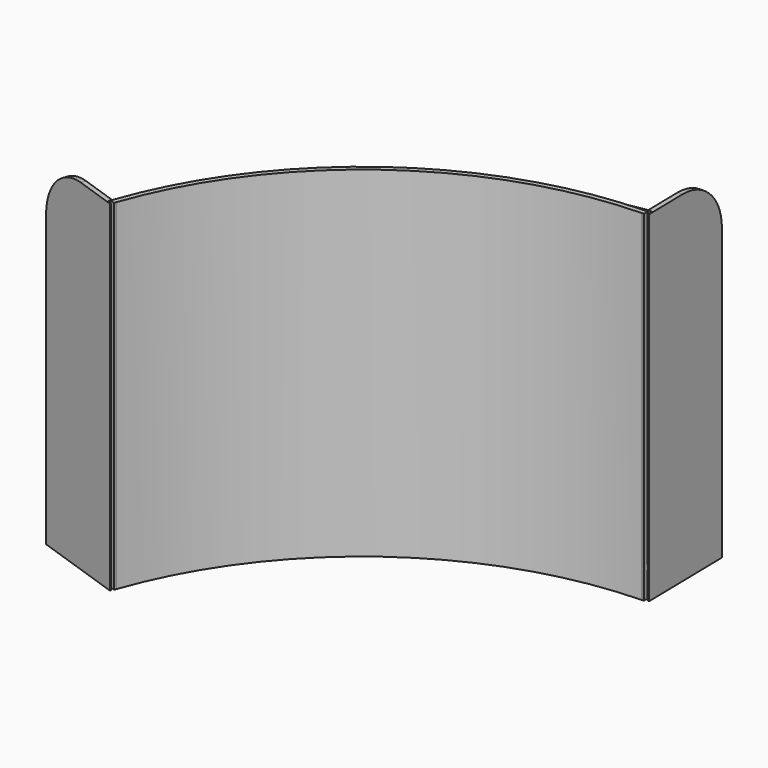
from build123d import *

# Parameters (mm, degrees)
F1_DEPTH  = 19.558
F0_R      = 2.499995
F3_DEPTH  = 19.558
F6_W      = 317.5
F6_H      = 19.558
F6_W_2    = 19.558
F6_H_2    = 1250.442
F6_H_3    = 101.6
F11_DEPTH = 19.558
F12_DEPTH = 6.35
F13_DEPTH = 15.875
F15_DEPTH = 1371.6


with BuildPart() as f1:
    # F0 (on Top) → F1 (new body)
    with BuildSketch(Plane.XY):
        with BuildLine():
            Line((-38.3338824503, 1504.9698678779), (-44.5220498384, 1828.257976074))
            ThreePointArc((-44.5220498384, 1828.257976074), (-1077.4341988171, 1477.7161389182), (-1727.0562659603, 601.4865702635))
            Line((-1727.0562659603, 601.4865702635), (-1421.1483384022, 496.730500393))
            ThreePointArc((-1421.1483384022, 496.730500393), (-886.9378466289, 1216.4477160903), (-38.3338824504, 1504.9698678779))
        make_face()
    extrude(amount=F1_DEPTH)


with BuildPart() as f1_1:
    # F2: moved
    add(f1.part.moved(Location((0, 0, 508))))


with BuildPart() as f3:
    # F0 (on Top) → F3 (new body)
    with BuildSketch(Plane.XY):
        with BuildLine():
            Line((-38.3338824503, 1504.9698678779), (-44.5220498384, 1828.257976074))
            ThreePointArc((-44.5220498384, 1828.257976074), (-1077.4341988171, 1477.7161389182), (-1727.0562659603, 601.4865702635))
            Line((-1727.0562659603, 601.4865702635), (-1421.1483384022, 496.730500393))
            ThreePointArc((-1421.1483384022, 496.730500393), (-886.9378466289, 1216.4477160903), (-38.3338824504, 1504.9698678779))
        make_face()
        with BuildLine():
            ThreePointArc((-1727.0562659603, 601.4865702635), (-1727.5777439387, 599.9871487356), (-1728.0979201271, 598.4872750964))
            Line((-1728.0979201271, 598.4872750964), (-1692.0632335536, 586.1474440414))
            Line((-1692.0632335536, 586.1474440414), (-1422.1927927873, 493.7321641415))
            ThreePointArc((-1422.1927927873, 493.7321641415), (-1421.6713560396, 495.2316076145), (-1421.1483384022, 496.730500393))
            Line((-1421.1483384022, 496.730500393), (-1727.0562659603, 601.4865702635))
        make_face()
        with BuildLine():
            Line((-1692.0632335536, 586.1474440414), (-1694.1204673289, 580.1399246537))
            Line((-1694.1204673289, 580.1399246537), (-1424.2626964338, 487.7289834642))
            ThreePointArc((-1424.2626964338, 487.7289834642), (-1423.2309097873, 490.7316651594), (-1422.1927927873, 493.7321641415))
            Line((-1422.1927927873, 493.7321641415), (-1692.0632335536, 586.1474440414))
        make_face()
        with BuildLine():
            ThreePointArc((-1410.177646219, 489.6176596778), (-1411.2158440245, 486.6171884945), (-1412.2476576585, 483.6145159134))
            Line((-1412.2476576585, 483.6145159134), (-1393.7444979444, 477.2782358853))
            ThreePointArc((-1393.7444979444, 477.2782358852), (-1392.712641839, 480.2808941252), (-1391.6743168688, 483.2813215589))
            Line((-1391.6743168688, 483.2813215589), (-1410.177646219, 489.6176596778))
        make_face()
        with BuildLine():
            Line((-1390.6295156867, 486.2795390522), (-1409.1330570886, 492.6159497867))
            ThreePointArc((-1409.1330570885, 492.6159497867), (-1409.6561488115, 491.117082458), (-1410.177646219, 489.6176596778))
            Line((-1410.177646219, 489.6176596778), (-1391.6743168688, 483.2813215589))
            ThreePointArc((-1391.6743168688, 483.2813215589), (-1391.1527239992, 484.7807117756), (-1390.6295156867, 486.2795390523))
        make_face()
        with BuildLine():
            Line((-37.7165215831, 1472.7171160816), (-38.0908270559, 1492.2719375027))
            ThreePointArc((-38.090827056, 1492.2719375027), (-879.4556646891, 1206.1857984615), (-1409.1330570885, 492.6159497867))
            Line((-1409.1330570886, 492.6159497867), (-1390.6295156867, 486.2795390522))
            ThreePointArc((-1390.6295156867, 486.2795390523), (-867.9331045017, 1190.3824453133), (-37.7165215832, 1472.7171160816))
        make_face()
        with Locations((-1377.7010357899, 548.0997004273)):
            Circle(F0_R, mode=Mode.SUBTRACT)
        with Locations((-1297.8643706073, 716.9529281153)):
            Circle(F0_R, mode=Mode.SUBTRACT)
        with Locations((-1197.4332353353, 874.4295697994)):
            Circle(F0_R, mode=Mode.SUBTRACT)
        with Locations((-1078.0012679981, 1018.0307911943)):
            Circle(F0_R, mode=Mode.SUBTRACT)
        with Locations((-941.4636112121, 1145.4779327375)):
            Circle(F0_R, mode=Mode.SUBTRACT)
        with Locations((-789.9868401238, 1254.7486672861)):
            Circle(F0_R, mode=Mode.SUBTRACT)
        with Locations((-625.9745832649, 1344.1090903388)):
            Circle(F0_R, mode=Mode.SUBTRACT)
        with Locations((-452.0293818519, 1412.1412335767)):
            Circle(F0_R, mode=Mode.SUBTRACT)
        with Locations((-270.9113927464, 1457.7655651391)):
            Circle(F0_R, mode=Mode.SUBTRACT)
        with Locations((-85.4945903742, 1480.2581196)):
            Circle(F0_R, mode=Mode.SUBTRACT)
        with BuildLine():
            Line((-40.6188210058, 1790.2435390022), (-41.3478950533, 1828.3325166869))
            ThreePointArc((-41.3478950533, 1828.3325166869), (-42.9349886223, 1828.2959352227), (-44.5220498384, 1828.257976074))
            Line((-44.5220498384, 1828.257976074), (-38.3338824503, 1504.9698678779))
            ThreePointArc((-38.3338824504, 1504.9698678779), (-36.7468538116, 1505.0094546211), (-35.1597843105, 1505.0473678032))
            Line((-35.1597843105, 1505.0473678032), (-40.6188210058, 1790.2435390022))
        make_face()
        with BuildLine():
            Line((-28.811204863, 1505.182282728), (-34.2699852614, 1790.3650642217))
            Line((-34.2699852614, 1790.3650642217), (-40.6188210058, 1790.2435390022))
            Line((-40.6188210058, 1790.2435390022), (-35.1597843105, 1505.0473678032))
            ThreePointArc((-35.1597843105, 1505.0473678032), (-31.9855657206, 1505.1181725531), (-28.811204863, 1505.182282728))
        make_face()
        with BuildLine():
            Line((-28.1938566232, 1472.930190623), (-28.5681543749, 1492.4846086709))
            ThreePointArc((-28.5681543749, 1492.4846086709), (-31.742514808, 1492.4204700143), (-34.9167316418, 1492.3495798289))
            Line((-34.9167316418, 1492.3495798289), (-34.5424304585, 1472.7949825071))
            ThreePointArc((-34.5424304586, 1472.7949825071), (-31.3682163903, 1472.8660071441), (-28.1938566231, 1472.930190623))
        make_face()
        with BuildLine():
            ThreePointArc((-34.9167316418, 1492.3495798289), (-36.5037999917, 1492.311602565), (-38.090827056, 1492.2719375027))
            Line((-38.0908270559, 1492.2719375027), (-37.7165215831, 1472.7171160816))
            ThreePointArc((-37.7165215832, 1472.7171160816), (-36.1294969981, 1472.7569043962), (-34.5424304586, 1472.7949825071))
            Line((-34.5424304585, 1472.7949825071), (-34.9167316418, 1492.3495798289))
        make_face()
        with Locations((-1078.0012679981, 1018.0307911943)):
            Circle(F0_R)
        with Locations((-1297.8643706073, 716.9529281153)):
            Circle(F0_R)
        with Locations((-1197.4332353353, 874.4295697994)):
            Circle(F0_R)
        with Locations((-1377.7010357899, 548.0997004273)):
            Circle(F0_R)
        with Locations((-941.4636112121, 1145.4779327375)):
            Circle(F0_R)
        with Locations((-625.9745832649, 1344.1090903388)):
            Circle(F0_R)
        with Locations((-270.9113927464, 1457.7655651391)):
            Circle(F0_R)
        with Locations((-452.0293818519, 1412.1412335767)):
            Circle(F0_R)
        with Locations((-789.9868401238, 1254.7486672861)):
            Circle(F0_R)
        with Locations((-85.4945903742, 1480.2581196)):
            Circle(F0_R)
        with BuildLine():
            ThreePointArc((-1422.1927927873, 493.7321641415), (-1423.2309097873, 490.7316651594), (-1424.2626964338, 487.7289834642))
            Line((-1424.2626964338, 487.7289834642), (-1412.2476576585, 483.6145159134))
            ThreePointArc((-1412.2476576585, 483.6145159134), (-1411.2158440245, 486.6171884945), (-1410.177646219, 489.6176596778))
            Line((-1410.177646219, 489.6176596778), (-1422.1927927873, 493.7321641415))
        make_face()
        with BuildLine():
            Line((-1409.1330570886, 492.6159497867), (-1421.1483384022, 496.730500393))
            ThreePointArc((-1421.1483384022, 496.730500393), (-1421.6713560396, 495.2316076145), (-1422.1927927873, 493.7321641415))
            Line((-1422.1927927873, 493.7321641415), (-1410.177646219, 489.6176596778))
            ThreePointArc((-1410.177646219, 489.6176596778), (-1409.6561488115, 491.117082458), (-1409.1330570885, 492.6159497867))
        make_face()
        with BuildLine():
            Line((-38.0908270559, 1492.2719375027), (-38.3338824503, 1504.9698678779))
            ThreePointArc((-38.3338824504, 1504.9698678779), (-886.9378466289, 1216.4477160903), (-1421.1483384022, 496.730500393))
            Line((-1421.1483384022, 496.730500393), (-1409.1330570886, 492.6159497867))
            ThreePointArc((-1409.1330570885, 492.6159497867), (-879.4556646891, 1206.1857984615), (-38.090827056, 1492.2719375027))
        make_face()
        with BuildLine():
            ThreePointArc((-35.1597843105, 1505.0473678032), (-36.7468538116, 1505.0094546211), (-38.3338824504, 1504.9698678779))
            Line((-38.3338824503, 1504.9698678779), (-38.0908270559, 1492.2719375027))
            ThreePointArc((-38.090827056, 1492.2719375027), (-36.5037999917, 1492.311602565), (-34.9167316418, 1492.3495798289))
            Line((-34.9167316418, 1492.3495798289), (-35.1597843105, 1505.0473678032))
        make_face()
        with BuildLine():
            Line((-28.5681543749, 1492.4846086709), (-28.811204863, 1505.182282728))
            ThreePointArc((-28.811204863, 1505.182282728), (-31.9855657206, 1505.1181725531), (-35.1597843105, 1505.0473678032))
            Line((-35.1597843105, 1505.0473678032), (-34.9167316418, 1492.3495798289))
            ThreePointArc((-34.9167316418, 1492.3495798289), (-31.742514808, 1492.4204700143), (-28.5681543749, 1492.4846086709))
        make_face()
    extrude(amount=-F3_DEPTH)


with BuildPart() as f4_1:
    # F4: copy of F1
    add(f1_1.part.moved(Location((0, 0, 381))))


with BuildPart() as f5_1:
    # F5: copy of F4_1
    add(f4_1.part.moved(Location((0, 0, 381))))


with BuildPart() as f1_2:
    # F7: moved
    add(f1_1.part.moved(Location((0, 0, -127))))


with BuildPart() as f4_1_1:
    # F8: moved
    add(f4_1.part.moved(Location((0, 0, -203.2))))


with BuildPart() as f1_3:
    # F9: moved
    add(f1_2.part.moved(Location((0, 0, -50.8))))


with BuildPart() as f5_1_1:
    # F10: moved
    add(f5_1.part.moved(Location((0, 0, -254))))


with BuildPart() as f11:
    # F6 (on face) → F11 (new body)
    with BuildSketch(Plane(origin=(0, 0, 0), x_dir=(0.9460660453, -0.3239738229, 0), z_dir=(-0.3239738229, -0.9460660453, 0))):
        with Locations((-1631.95, -9.779)):
            Rectangle(F6_W, F6_H)
        with Locations((-1463.4099756612, 625.221)):
            Rectangle(F6_W_2, F6_H_2)
        with Locations((-1463.4099756612, -70.358)):
            Rectangle(F6_W_2, F6_H_3)
        with Locations((-1463.4099756612, -9.779)):
            Rectangle(F6_W_2, F6_H)
        with BuildLine():
            Line((-1828.7889756612, 1047.242), (-1828.7889756612, -121.158))
            Line((-1828.7889756612, -121.158), (-1473.1889756612, -121.158))
            Line((-1473.1889756612, -121.158), (-1473.1889756612, -19.558))
            Line((-1473.1889756612, -19.558), (-1473.2, -19.558))
            Line((-1473.2, -19.558), (-1790.7, -19.558))
            Line((-1790.7, -19.558), (-1790.7, 0))
            Line((-1790.7, 0), (-1473.2, 0))
            Line((-1473.2, 0), (-1473.1889756612, 0))
            Line((-1473.1889756612, 0), (-1473.1889756612, 1250.442))
            Line((-1473.1889756612, 1250.442), (-1625.5889756612, 1250.442))
            ThreePointArc((-1625.5889756612, 1250.442), (-1769.2730735983, 1190.9260979371), (-1828.7889756612, 1047.242))
        make_face()
        with Locations((-1631.95, -9.779)):
            Rectangle(F6_W, F6_H)
    extrude(amount=F11_DEPTH)

    # F6 (on face) → F12 (cut)
    with BuildSketch(Plane(origin=(0, 0, 0), x_dir=(0.9460660453, -0.3239738229, 0), z_dir=(-0.3239738229, -0.9460660453, 0))):
        with Locations((-1631.95, -9.779)):
            Rectangle(F6_W, F6_H)
    extrude(amount=F12_DEPTH, mode=Mode.SUBTRACT)

    # F6 (on face) → F13 (cut)
    with BuildSketch(Plane(origin=(0, 0, 0), x_dir=(0.9460660453, -0.3239738229, 0), z_dir=(-0.3239738229, -0.9460660453, 0))):
        with Locations((-1463.4099756612, 625.221)):
            Rectangle(F6_W_2, F6_H_2)
        with Locations((-1463.4099756612, -9.779)):
            Rectangle(F6_W_2, F6_H)
        with Locations((-1463.4099756612, -70.358)):
            Rectangle(F6_W_2, F6_H_3)
    extrude(amount=F13_DEPTH, mode=Mode.SUBTRACT)


with BuildPart() as f11_1:
    # F14: moved
    add(f11.part.moved(Location((0, 6.35, 0))))


with BuildPart() as f15:
    # F0 (on Top) → F15 (new body)
    with BuildSketch(Plane.XY):
        with BuildLine():
            ThreePointArc((-1391.6743168688, 483.2813215589), (-1392.712641839, 480.2808941252), (-1393.7444979444, 477.2782358852))
            Line((-1393.7444979444, 477.2782358853), (-1375.2413382303, 470.9419558572))
            ThreePointArc((-1375.2413382303, 470.9419558572), (-1374.2094385098, 473.9445993726), (-1373.1709829539, 476.9449818769))
            Line((-1373.1709829539, 476.9449818769), (-1391.6743168688, 483.2813215589))
        make_face()
        with BuildLine():
            Line((-1372.1259640138, 479.9431248005), (-1390.6295156867, 486.2795390522))
            ThreePointArc((-1390.6295156867, 486.2795390523), (-1391.1527239992, 484.7807117756), (-1391.6743168688, 483.2813215589))
            Line((-1391.6743168688, 483.2813215589), (-1373.1709829539, 476.9449818769))
            ThreePointArc((-1373.1709829539, 476.9449818769), (-1372.6492920527, 478.4443386553), (-1372.1259640138, 479.9431248004))
        make_face()
        with BuildLine():
            Line((-37.3422159025, 1453.1622838057), (-37.7165215831, 1472.7171160816))
            ThreePointArc((-37.7165215832, 1472.7171160816), (-867.9331045017, 1190.3824453133), (-1390.6295156867, 486.2795390523))
            Line((-1390.6295156867, 486.2795390522), (-1372.1259640138, 479.9431248005))
            ThreePointArc((-1372.1259640138, 479.9431248004), (-856.4105443144, 1174.579092165), (-37.3422159025, 1453.1622838057))
        make_face()
        with BuildLine():
            ThreePointArc((-34.5424304586, 1472.7949825071), (-36.1294969981, 1472.7569043962), (-37.7165215832, 1472.7171160816))
            Line((-37.7165215831, 1472.7171160816), (-37.3422159025, 1453.1622838057))
            ThreePointArc((-37.3422159025, 1453.1622838057), (-35.7551938651, 1453.2021986894), (-34.168129183, 1453.2403803611))
            Line((-34.1681291829, 1453.2403803611), (-34.5424304585, 1472.7949825071))
        make_face()
        with BuildLine():
            Line((-27.8195588714, 1453.3757725751), (-28.1938566232, 1472.930190623))
            ThreePointArc((-28.1938566231, 1472.930190623), (-31.3682163903, 1472.8660071441), (-34.5424304586, 1472.7949825071))
            Line((-34.5424304585, 1472.7949825071), (-34.1681291829, 1453.2403803611))
            ThreePointArc((-34.168129183, 1453.2403803611), (-30.9939179573, 1453.3115430676), (-27.8195588715, 1453.3757725751))
        make_face()
    extrude(amount=F15_DEPTH)


with BuildPart() as f15_1:
    # F16: moved
    add(f15.part.moved(Location((0, 0, -101.6))))


with BuildPart() as f15_2:
    # F17: moved
    add(f15_1.part.moved(Location((0, 0, -19.05))))


with BuildPart() as f19_1:
    # F19: instance of F11
    add(f11_1.part.mirror(Plane(origin=(-378.298980069, 527.6714093386, 127), x_dir=(-0.5891481842, 0.8080250101, 0), z_dir=(0.8080250101, 0.5891481842, 0))))


with BuildPart() as f19_1_1:
    # F21: moved
    add(f19_1.part.moved(Location((-7.62, 0, 0))))


solid = Compound([f3.part, f4_1_1.part, f1_3.part, f5_1_1.part, f11_1.part, f15_2.part, f19_1_1.part])
